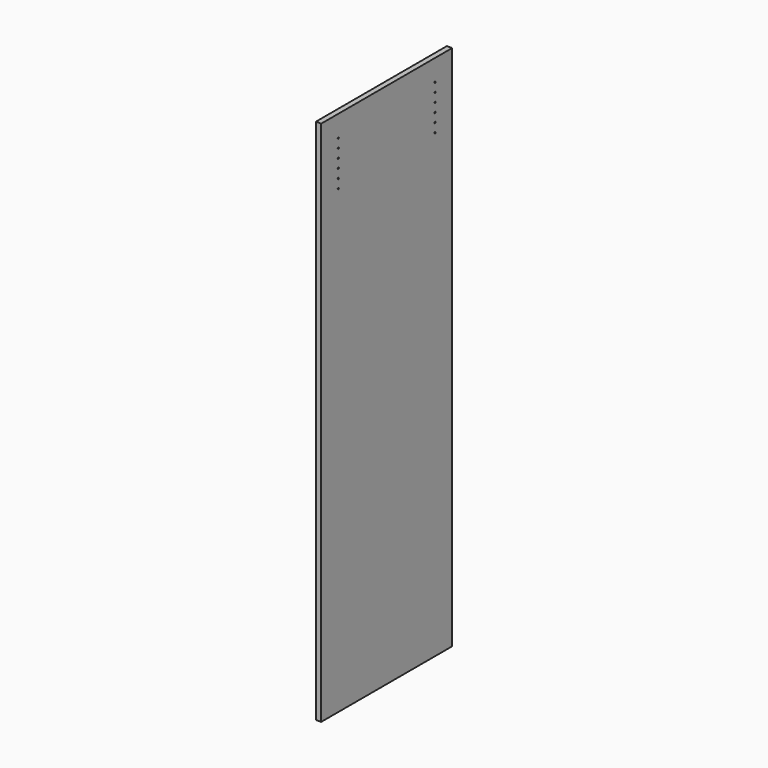
from build123d import *

# Parameters (mm, degrees)
F0_W     = 584.2
F0_H     = 1879.6
F1_DEPTH = 19.05
F3_D     = 5.0038
F3_DEPTH = 14.224
F3_TIP   = 1.5032931827


# Not quite as in the source:
# - a feature names something its author has since deleted; it is built from what else it names


with BuildPart() as f1:
    # F0 (on Right) → F1 (new body)
    with BuildSketch(Plane.YZ):
        Rectangle(F0_W, F0_H)
    extrude(amount=F1_DEPTH)

    # F3
    with Locations(Plane.YZ.offset(19.05)):
        with Locations((-215.9, 863.6), (-215.9, 831.85), (-215.9, 800.1), (-215.9, 768.35), (-215.9, 736.6), (215.9, 863.6), (215.9, 831.85), (215.9, 800.1), (215.9, 768.35), (215.9, 736.6), (-215.9, 704.85), (215.9, 704.85)):
            Hole(F3_D / 2, depth=F3_DEPTH)
            with Locations((0, 0, -(F3_DEPTH + F3_TIP / 2))):  # 118° drill point
                Cone(0, F3_D / 2, F3_TIP, mode=Mode.SUBTRACT)


solid = f1.part
